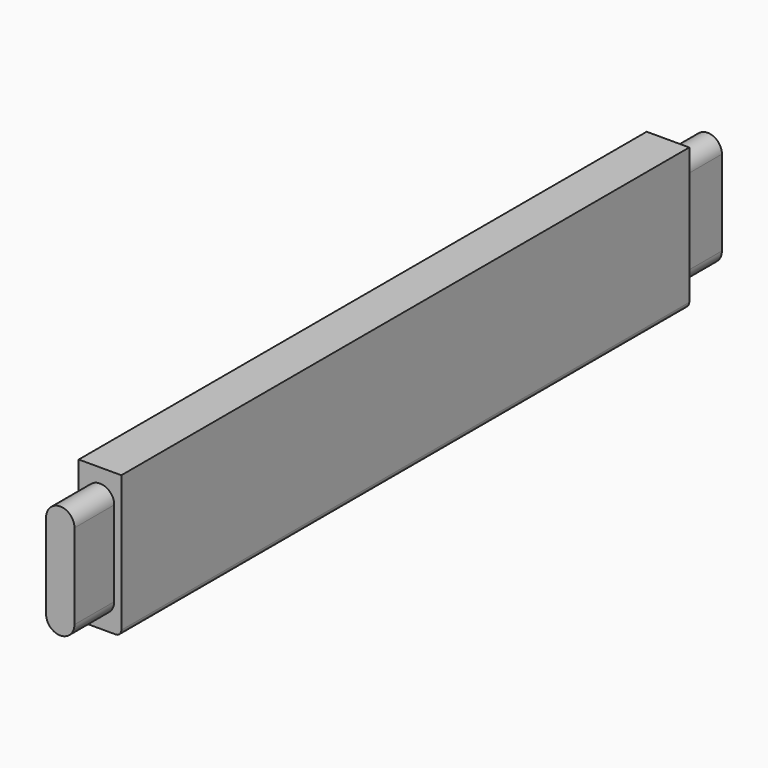
from build123d import *

# Parameters (mm, degrees)
F0_W          = 15
F0_H          = 50
F1_DEPTH      = 142.5
F1_DEPTH_BACK = 142.5
F2_W          = 15
F2_H          = 50
F3_DEPTH      = 17.5
F4_R          = 2


# Not quite as in the source:
# - a pattern or mirror of a feature is missing from the dataset's text; its kind, count and spacing are read off the source's solid


with BuildPart() as f1:
    # F0 (on Front) → F1 (new body, two sides)
    with BuildSketch(Plane.XZ) as f1_sk:
        Rectangle(F0_W, F0_H)
    extrude(amount=F1_DEPTH)
    extrude(f1_sk.sketch, amount=-F1_DEPTH_BACK)

    # F2 (on face) → F3 (cut)
    with BuildSketch(Plane.XZ.offset(142.5)):
        Rectangle(F2_W, F2_H)
        with BuildLine():
            ThreePointArc((5, -15), (0, -20), (-5, -15))
            Line((-5, -15), (-5, 15))
            ThreePointArc((-5, 15), (0, 20), (5, 15))
            Line((5, 15), (5, -15))
        make_face(mode=Mode.SUBTRACT)
    f3 = extrude(amount=-F3_DEPTH, mode=Mode.SUBTRACT)

    # F3_copies: F3 across plane
    add(f3.mirror(Plane.ZX), mode=Mode.SUBTRACT)

    # F4
    f4_edges = [f1.edges().sort_by_distance(p)[0] for p in [
        (7.5, 0, -25),
        (-7.5, 0, -25),
    ]]
    fillet(f4_edges, radius=F4_R)


solid = f1.part
